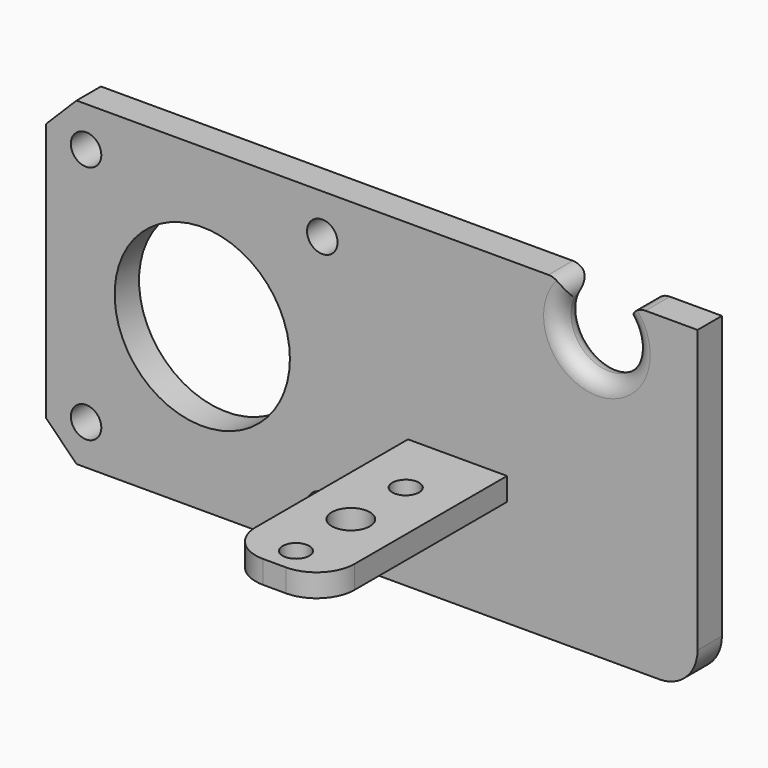
from build123d import *

# Parameters (mm, degrees)
F0_W      = 63.5
F0_H      = 42
F0_R      = 2
F0_R_2    = 11.5
F1_DEPTH  = 4
F2_SIZE   = 4
F3_W      = 13
F3_H      = 3
F4_DEPTH  = 30
F5_R      = 5
F6_R      = 2.5
F6_R_2    = 1.75
F7_DEPTH  = 3
F8_W      = 4
F8_H      = 42
F9_DEPTH  = 22
F10_R     = 5
F11_R     = 5
F12_DEPTH = 4
F13_R     = 1.99999


# Not quite as in the source:
# - a fillet or chamfer is up to 0.001 mm smaller than in the source, because OpenCascade refuses the exact size


with BuildPart() as f1:
    # F0 (on Front) → F1 (new body)
    with BuildSketch(Plane.XZ):
        with Locations((11.25, -0.25)):
            Rectangle(F0_W, F0_H)
        with Locations((-15.25, -16)):
            Circle(F0_R, mode=Mode.SUBTRACT)
        with Locations((15.75, -16)):
            Circle(F0_R, mode=Mode.SUBTRACT)
        Circle(F0_R_2, mode=Mode.SUBTRACT)
        with Locations((-15.25, 15.5)):
            Circle(F0_R, mode=Mode.SUBTRACT)
        with Locations((15.75, 15.5)):
            Circle(F0_R, mode=Mode.SUBTRACT)
    extrude(amount=F1_DEPTH)

    # F2
    f2_edges = [f1.edges().sort_by_distance(p)[0] for p in [
        (-20.5, -2, -21.25),
        (-20.5, -2, 20.75),
    ]]
    chamfer(f2_edges, length=F2_SIZE)

    # F3 (on face) → F4 (join)
    with BuildSketch(Plane.XZ.offset(4)):
        with Locations((33.5, -5.75)):
            Rectangle(F3_W, F3_H)
    extrude(amount=F4_DEPTH)

    # F5
    f5_edges = [f1.edges().sort_by_distance(p)[0] for p in [
        (40, -34, -5.75),
        (27, -34, -5.75),
    ]]
    fillet(f5_edges, radius=F5_R)

    # F6 (on face) → F7 (cut, through all)
    with BuildSketch(Plane.XY.offset(-4.25)):
        with Locations((33.5, -21.5)):
            Circle(F6_R)
        with Locations((33.5, -30.5)):
            Circle(F6_R_2)
        with Locations((33.5, -12.5)):
            Circle(F6_R_2)
    extrude(amount=-F7_DEPTH, mode=Mode.SUBTRACT)

    # F8 (on face) → F9 (join)
    with BuildSketch(Plane.YZ.offset(43)):
        with Locations((-2, -0.25)):
            Rectangle(F8_W, F8_H)
    extrude(amount=F9_DEPTH)

    # F10
    f10_edges = [f1.edges().sort_by_distance(p)[0] for p in [
        (65, -2, -21.25),
    ]]
    fillet(f10_edges, radius=F10_R)

    # F11 (on face) → F12 (cut, through all)
    with BuildSketch(Plane.XZ.offset(4)):
        with Locations((51.7936311662, 15.85)):
            Circle(F11_R)
    extrude(amount=-F12_DEPTH, mode=Mode.SUBTRACT)

    # F13 (radius 2 in the source; OpenCascade refuses exactly that, so slightly less here)
    f13_edges = [f1.edges().sort_by_distance(p)[0] for p in [
        (51.793631, -4, 10.85),
        (51.793631, 0, 10.85),
        (50.798644, -2, 20.75),
        (52.788619, -2, 20.75),
    ]]
    fillet(f13_edges, radius=F13_R)


solid = f1.part
